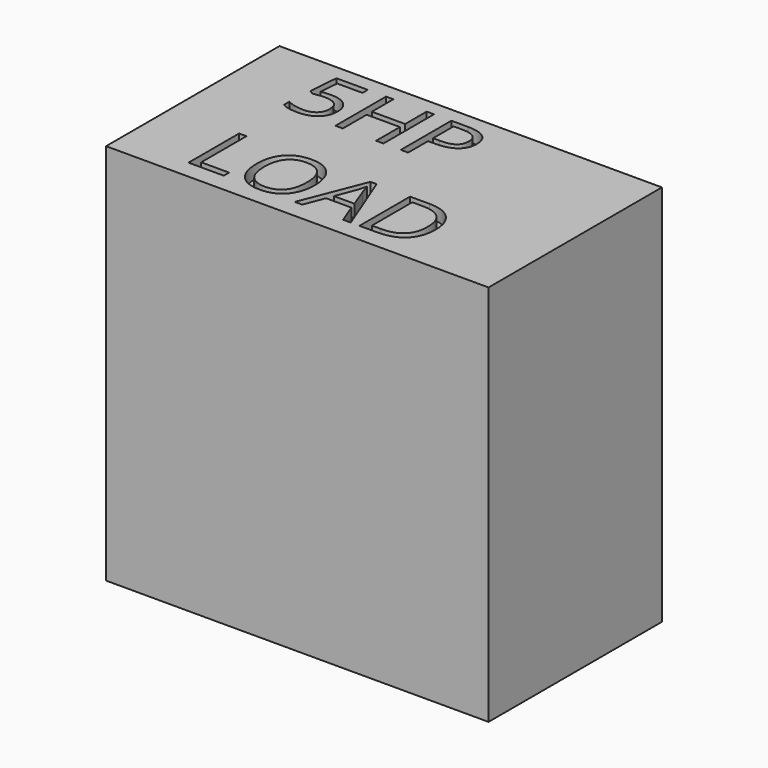
from build123d import *

# Parameters (mm, degrees)
F0_W         = 152.4
F0_H         = 86.36
F1_DEPTH     = 152.4
F2_TEXT_SIZE = 35.2777777778
F3_DEPTH     = 5


# Not quite as in the source:
# - Text() gives the source's letters only with a copy of the font that has no kerning and outlines rounded to 1/6400 em; it was checked with that copy


with BuildPart() as f1:
    # F0 (on Top) → F1 (new body)
    with BuildSketch(Plane.XY):
        Rectangle(F0_W, F0_H)
    extrude(amount=F1_DEPTH)

    # F2 (on face) → F3 (cut)
    with BuildSketch(Plane.XY.offset(152.4)):
        with Locations((-52.6840654536, 12.1474420581)):
            Text('5HP', F2_TEXT_SIZE, font='Open Sans', text_align=(TextAlign.LEFT, TextAlign.BOTTOM))
        with Locations((-52.6840654536, -35.8303357197)):
            Text('LOAD', F2_TEXT_SIZE, font='Open Sans', text_align=(TextAlign.LEFT, TextAlign.BOTTOM))
    extrude(amount=-F3_DEPTH, mode=Mode.SUBTRACT)


solid = f1.part
